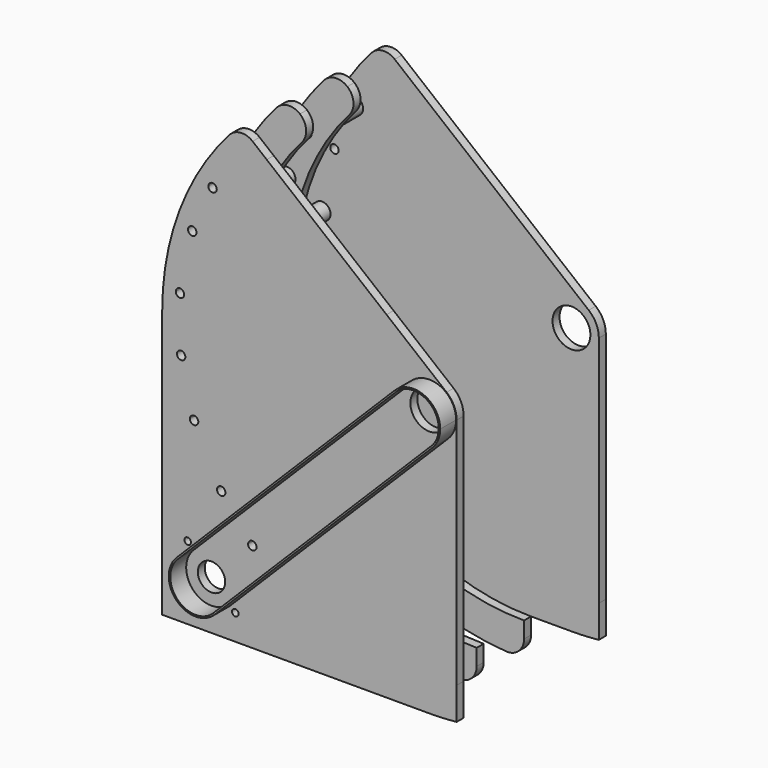
from build123d import *
from build123d import SkipClean  # not in build123d's __all__

# Parameters (mm, degrees)
F0_R      = 3.175
F0_R_2    = 2.4892
F0_R_3    = 19.1008
F0_R_4    = 10.31875
F1_DEPTH  = 6.604
F2_R      = 6.35
F3_DEPTH  = 38.1
F4_R      = 6.35
F4_R_2    = 3.175
F5_DEPTH  = 6.604
F6_R      = 6.35
F7_DEPTH  = 38.1
F8_R      = 3.175
F9_DEPTH  = 6.604
F10_R     = 6.35
F11_DEPTH = 38.1
F12_R     = 3.175
F12_R_2   = 25.4
F12_R_3   = 14.2875
F13_DEPTH = 6.604
F14_R     = 3.175
F15_DEPTH = 140.717
F16_R     = 12.69999
F18_DEPTH = 15


# Not quite as in the source:
# - a fillet or chamfer is up to 0.001 mm smaller than in the source, because OpenCascade refuses the exact size


with BuildPart() as f1:
    # F0 (on Front) → F1 (new body)
    with BuildSketch(Plane.XZ):
        with BuildLine():
            Line((20.6375, -174.9998249999), (20.6375, -58.3716647869))
            ThreePointArc((20.6375, -58.3716647869), (-52.3694193672, -33.0242573178), (-43.7787485902, 43.7787485902))
            Line((-43.7787485902, 43.7787485902), (-124.6010536798, 124.6010536798))
            ThreePointArc((-124.6010536798, 124.6010536798), (-162.7991221226, -67.4336043256), (0, -176.2125))
            ThreePointArc((0, -176.2125), (10.3365490724, -175.9090700036), (20.6375, -174.9998249999))
        make_face()
        with BuildLine():
            ThreePointArc((0, -176.2125), (-162.7991221226, -67.4336043256), (-124.6010536798, 124.6010536798))
            Line((-124.6010536798, 124.6010536798), (-142.561565922, 142.561565922))
            ThreePointArc((-142.561565922, 142.561565922), (-186.2656622484, 77.1537635077), (-201.6125, 0))
            ThreePointArc((-201.6125, 0), (-172.0465507714, -105.1074903321), (-92.0202423383, -179.3875))
            Line((-92.0202423383, -179.3875), (20.6358525902, -179.3875))
            Line((20.6358525902, -179.3875), (20.6358525902, -176.2125))
            Line((20.6358525902, -176.2125), (0, -176.2125))
        make_face()
        with Locations((-133.5813098009, -133.5813098009)):
            Circle(F0_R, mode=Mode.SUBTRACT)
        with Locations((-177.5196822242, -64.611880326)):
            Circle(F0_R, mode=Mode.SUBTRACT)
        with Locations((-188.1936309033, 16.4648092518)):
            Circle(F0_R, mode=Mode.SUBTRACT)
        with Locations((-163.6030240924, 94.45625)):
            Circle(F0_R, mode=Mode.SUBTRACT)
        with BuildLine():
            ThreePointArc((-92.0202423383, -179.3875), (-172.0465507714, -105.1074903321), (-201.6125, 0))
            Line((-201.6125, 0), (-201.6125, -201.6125))
            Line((-201.6125, -201.6125), (0, -201.6125))
            ThreePointArc((0, -201.6125), (-47.3330635629, -195.9775018975), (-92.0202423383, -179.3875))
        make_face()
        with Locations((-146.444987879, -182.3660123632)):
            Circle(F0_R_2, mode=Mode.SUBTRACT)
        with Locations((-164.4055001211, -164.4055001211)):
            Circle(F0_R_3, mode=Mode.SUBTRACT)
        with Locations((-182.3660123632, -146.444987879)):
            Circle(F0_R_2, mode=Mode.SUBTRACT)
        with BuildLine():
            ThreePointArc((-43.7787485902, 43.7787485902), (-52.3694193672, -33.0242573178), (20.6375, -58.3716647869))
            Line((20.6375, -58.3716647869), (20.6375, 0))
            ThreePointArc((20.6375, 0), (-7.8976293354, -19.0665638522), (-14.5929161967, 14.5929161967))
            Line((-14.5929161967, 14.5929161967), (-43.7787485902, 43.7787485902))
        make_face()
        with BuildLine():
            Line((20.6358525902, -179.3875), (-92.0202423383, -179.3875))
            ThreePointArc((-92.0202423383, -179.3875), (-47.3330635629, -195.9775018975), (0, -201.6125))
            ThreePointArc((0, -201.6125), (10.3315003836, -201.347610505), (20.6358525902, -200.5536380725))
            Line((20.6358525902, -200.5536380725), (20.6358525902, -179.3875))
        make_face()
        with BuildLine():
            ThreePointArc((20.6375, 0), (18.6367679163, 8.864383108), (13.0224993569, 16.0100255074))
            ThreePointArc((13.0224993569, 16.0100255074), (-1.0576398075, 20.6103809836), (-14.5929161967, 14.5929161967))
            ThreePointArc((-14.5929161967, 14.5929161967), (-7.8976293354, -19.0665638522), (20.6375, 0))
        make_face()
        with BuildLine():
            ThreePointArc((19.1008, 0), (-7.3095597049, -17.6468381746), (-13.5063052061, 13.5063052061))
            ThreePointArc((-13.5063052061, 13.5063052061), (7.3095597049, 17.6468381746), (19.1008, 0))
        make_face(mode=Mode.SUBTRACT)
        with BuildLine():
            ThreePointArc((19.1008, 0), (7.3095597049, 17.6468381746), (-13.5063052061, 13.5063052061))
            ThreePointArc((-13.5063052061, 13.5063052061), (-7.3095597049, -17.6468381746), (19.1008, 0))
        make_face()
        with BuildLine():
            ThreePointArc((14.2875, 0), (-5.4675895399, -13.1999288208), (-10.1027881362, 10.1027881362))
            ThreePointArc((-10.1027881362, 10.1027881362), (5.4675895399, 13.1999288208), (14.2875, 0))
        make_face(mode=Mode.SUBTRACT)
        with Locations((-164.4055001211, -164.4055001211)):
            Circle(F0_R_3)
        with Locations((-164.4055001211, -164.4055001211)):
            Circle(F0_R_4, mode=Mode.SUBTRACT)
        with BuildLine():
            ThreePointArc((-43.7787485902, 43.7787485902), (-38.2889048868, 48.6530309315), (-32.2606910562, 52.8432159206))
            Line((-32.2606910562, 52.8432159206), (-122.7377265448, 126.4369235582))
            ThreePointArc((-122.7377265448, 126.4369235582), (-123.6727967473, 125.5224462037), (-124.6010536798, 124.6010536798))
            Line((-124.6010536798, 124.6010536798), (-43.7787485902, 43.7787485902))
        make_face()
        with BuildLine():
            Line((13.0224993569, 16.0100255074), (-32.2606910562, 52.8432159206))
            ThreePointArc((-32.2606910562, 52.8432159206), (-38.2889048868, 48.6530309315), (-43.7787485902, 43.7787485902))
            Line((-43.7787485902, 43.7787485902), (-14.5929161967, 14.5929161967))
            ThreePointArc((-14.5929161967, 14.5929161967), (-1.0576398075, 20.6103809836), (13.0224993569, 16.0100255074))
        make_face()
        with BuildLine():
            ThreePointArc((-124.6010536798, 124.6010536798), (-123.6727967473, 125.5224462037), (-122.7377265448, 126.4369235582))
            Line((-122.7377265448, 126.4369235582), (-142.561565922, 142.561565922))
            Line((-142.561565922, 142.561565922), (-124.6010536798, 124.6010536798))
        make_face()
        with BuildLine():
            Line((20.6375, -176.2125), (20.6375, -174.9998249999))
            ThreePointArc((20.6375, -174.9998249999), (10.3365490724, -175.9090700036), (0, -176.2125))
            Line((0, -176.2125), (20.6358525902, -176.2125))
            Line((20.6358525902, -176.2125), (20.6375, -176.2125))
        make_face()
    extrude(amount=F1_DEPTH)

    # F2 (on face) → F3 (join)
    with BuildSketch(Plane(origin=(0, 0, 0), x_dir=(-1, 0, 0), z_dir=(0, 1, 0))):
        with Locations((163.6030240924, 94.45625)):
            Circle(F2_R)
        with Locations((188.1936309033, 16.4648092518)):
            Circle(F2_R)
        with Locations((177.5196822242, -64.611880326)):
            Circle(F2_R)
        with Locations((133.5813098009, -133.5813098009)):
            Circle(F2_R)
    extrude(amount=F3_DEPTH)

    # F4 (on face) → F5 (join)
    with BuildSketch(Plane(origin=(0, 38.1, 0), x_dir=(-1, 0, 0), z_dir=(0, 1, 0))):
        with BuildLine():
            ThreePointArc((0, -201.6125), (142.561565922, -142.561565922), (201.6125, 0))
            ThreePointArc((201.6125, 0), (186.2656622484, 77.1537635077), (142.561565922, 142.561565922))
            Line((142.561565922, 142.561565922), (137.5828187691, 138.5118702131))
            ThreePointArc((137.5828187691, 138.5118702131), (139.3142009541, 136.3119615594), (139.9313098009, 133.5813098009))
            ThreePointArc((139.9313098009, 133.5813098009), (135.0804626561, 127.410812194), (127.9391709925, 130.6677604763))
            Line((127.9391709925, 130.6677604763), (122.7377265448, 126.4369235582))
            ThreePointArc((122.7377265448, 126.4369235582), (162.2941261953, 68.6400885689), (176.2125, 0))
            ThreePointArc((176.2125, 0), (124.6010536798, -124.6010536798), (0, -176.2125))
            Line((0, -176.2125), (0, -201.6125))
        make_face()
        with Locations((94.45625, -163.6030240924)):
            Circle(F4_R, mode=Mode.SUBTRACT)
        with Locations((133.5813098009, -133.5813098009)):
            Circle(F4_R_2, mode=Mode.SUBTRACT)
        with Locations((157.0750031341, -104.9541616453)):
            Circle(F4_R, mode=Mode.SUBTRACT)
        with Locations((177.5196822242, -64.611880326)):
            Circle(F4_R_2, mode=Mode.SUBTRACT)
        with Locations((187.2963273743, -24.6580292878)):
            Circle(F4_R, mode=Mode.SUBTRACT)
        with Locations((188.1936309033, 16.4648092518)):
            Circle(F4_R_2, mode=Mode.SUBTRACT)
        with Locations((178.8869380882, 60.7239329891)):
            Circle(F4_R, mode=Mode.SUBTRACT)
        with Locations((163.6030240924, 94.45625)):
            Circle(F4_R, mode=Mode.SUBTRACT)
        with BuildLine():
            ThreePointArc((139.9313098009, 133.5813098009), (139.3142009541, 136.3119615594), (137.5828187691, 138.5118702131))
            Line((137.5828187691, 138.5118702131), (127.9391709925, 130.6677604763))
            ThreePointArc((127.9391709925, 130.6677604763), (135.0804626561, 127.410812194), (139.9313098009, 133.5813098009))
        make_face()
        with Locations((178.8869380882, 60.7239329891)):
            Circle(F4_R)
        with Locations((178.8869380882, 60.7239329891)):
            Circle(F4_R_2, mode=Mode.SUBTRACT)
        with Locations((187.2963273743, -24.6580292878)):
            Circle(F4_R)
        with Locations((187.2963273743, -24.6580292878)):
            Circle(F4_R_2, mode=Mode.SUBTRACT)
        with Locations((157.0750031341, -104.9541616453)):
            Circle(F4_R)
        with Locations((157.0750031341, -104.9541616453)):
            Circle(F4_R_2, mode=Mode.SUBTRACT)
        with Locations((94.45625, -163.6030240924)):
            Circle(F4_R)
        with Locations((163.6030240924, 94.45625)):
            Circle(F4_R)
        with Locations((163.6030240924, 94.45625)):
            Circle(F4_R_2, mode=Mode.SUBTRACT)
    extrude(amount=F5_DEPTH)

    # F6 (on face) → F7 (join)
    with BuildSketch(Plane(origin=(0, 44.704, 0), x_dir=(-1, 0, 0), z_dir=(0, 1, 0))):
        with Locations((178.8869380882, 60.7239329891)):
            Circle(F6_R)
        with Locations((187.2963273743, -24.6580292878)):
            Circle(F6_R)
        with Locations((157.0750031341, -104.9541616453)):
            Circle(F6_R)
    extrude(amount=F7_DEPTH)

    # F8 (on face) → F9 (join)
    with BuildSketch(Plane(origin=(0, 82.804, 0), x_dir=(-1, 0, 0), z_dir=(0, 1, 0))):
        with BuildLine():
            ThreePointArc((122.7377265448, 126.4369235582), (163.2951492678, -66.2234050912), (0, -176.2125))
            Line((0, -176.2125), (0, -201.6125))
            ThreePointArc((0, -201.6125), (186.2656622484, -77.1537635077), (142.561565922, 142.561565922))
            Line((142.561565922, 142.561565922), (122.7377265448, 126.4369235582))
        make_face()
        with Locations((133.5813098009, -133.5813098009)):
            Circle(F8_R, mode=Mode.SUBTRACT)
        with Locations((157.0750031341, -104.9541616453)):
            Circle(F8_R, mode=Mode.SUBTRACT)
        with Locations((177.5196822242, -64.611880326)):
            Circle(F8_R, mode=Mode.SUBTRACT)
        with Locations((187.2963273743, -24.6580292878)):
            Circle(F8_R, mode=Mode.SUBTRACT)
        with Locations((188.1936309033, 16.4648092518)):
            Circle(F8_R, mode=Mode.SUBTRACT)
        with Locations((163.6030240924, 94.45625)):
            Circle(F8_R, mode=Mode.SUBTRACT)
        with Locations((178.8869380882, 60.7239329891)):
            Circle(F8_R, mode=Mode.SUBTRACT)
    extrude(amount=F9_DEPTH)

    # F10 (on face) → F11 (join)
    with BuildSketch(Plane(origin=(0, 89.408, 0), x_dir=(-1, 0, 0), z_dir=(0, 1, 0))):
        with Locations((163.6030240924, 94.45625)):
            Circle(F10_R)
        with Locations((188.1936309033, 16.4648092518)):
            Circle(F10_R)
        with Locations((177.5196822242, -64.611880326)):
            Circle(F10_R)
        with Locations((133.5813098009, -133.5813098009)):
            Circle(F10_R)
    extrude(amount=F11_DEPTH)

    # F12 (on face) → F13 (join)
    with BuildSketch(Plane(origin=(0, 127.508, 0), x_dir=(-1, 0, 0), z_dir=(0, 1, 0))):
        with BuildLine():
            Line((142.561565922, 142.561565922), (-13.0224993569, 16.0100255074))
            ThreePointArc((-13.0224993569, 16.0100255074), (-18.6367679163, 8.864383108), (-20.6375, 0))
            Line((-20.6375, 0), (-20.6375, -176.2125))
            Line((-20.6375, -176.2125), (-20.6358525902, -200.5536380725))
            ThreePointArc((-20.6358525902, -200.5536380725), (-10.3315003836, -201.347610505), (0, -201.6125))
            Line((0, -201.6125), (201.6125, -201.6125))
            Line((201.6125, -201.6125), (201.6125, 0))
            ThreePointArc((201.6125, 0), (186.2656622484, 77.1537635077), (142.561565922, 142.561565922))
        make_face()
        with Locations((133.5813098009, -133.5813098009)):
            Circle(F12_R, mode=Mode.SUBTRACT)
        with Locations((164.4055001211, -164.4055001211)):
            Circle(F12_R_2, mode=Mode.SUBTRACT)
        with Locations((177.5196822242, -64.611880326)):
            Circle(F12_R, mode=Mode.SUBTRACT)
        Circle(F12_R_3, mode=Mode.SUBTRACT)
        with Locations((188.1936309033, 16.4648092518)):
            Circle(F12_R, mode=Mode.SUBTRACT)
        with Locations((163.6030240924, 94.45625)):
            Circle(F12_R, mode=Mode.SUBTRACT)
    extrude(amount=F13_DEPTH)

    # F14 (on face) → F15 (cut, through all)
    with BuildSketch(Plane(origin=(0, 134.112, 0), x_dir=(-1, 0, 0), z_dir=(0, 1, 0))):
        with Locations((163.6030240924, 94.45625)):
            Circle(F14_R)
        with Locations((188.1936309033, 16.4648092518)):
            Circle(F14_R)
        with Locations((177.5196822242, -64.611880326)):
            Circle(F14_R)
        with Locations((133.5813098009, -133.5813098009)):
            Circle(F14_R)
        with Locations((157.0750031341, -104.9541616453)):
            Circle(F14_R)
        with Locations((187.2963273743, -24.6580292878)):
            Circle(F14_R)
        with Locations((178.8869380882, 60.7239329891)):
            Circle(F14_R)
    with SkipClean():  # cleaning this boolean's faces spoils the solid; the shape is the same uncleaned
        extrude(amount=-F15_DEPTH, mode=Mode.SUBTRACT)

    # F16 (radius 12.7 in the source; OpenCascade refuses exactly that, so slightly less here)
    f16_edges = [f1.edges().sort_by_distance(p)[0] for p in [
        (-142.561566, -3.302, 142.561566),
        (-142.561566, 41.402, 142.561566),
        (-122.737727, 86.106, 126.436924),
        (-142.561566, 86.106, 142.561566),
        (-122.737727, 41.402, 126.436924),
        (-142.561566, 130.81, 142.561566),
        (0, 41.402, -201.6125),
        (0, 86.106, -201.6125),
    ]]
    fillet(f16_edges, radius=F16_R)


with BuildPart() as f18:
    # F17 (on face) → F18 (new body)
    with BuildSketch(Plane.XZ.offset(6.604)):
        with BuildLine():
            ThreePointArc((-14.314528257, 12.6465347594), (6.7609769749, 17.8642030605), (19.1008, 0))
            ThreePointArc((19.1008, 0), (17.4126317909, -7.8511664582), (12.6465347594, -14.314528257))
            Line((12.6465347594, -14.314528257), (8.6658675036, -18.2951955128))
            ThreePointArc((8.6658675036, -18.2951955128), (11.6613067569, -16.5476694178), (14.314528257, -14.314528257))
            ThreePointArc((14.314528257, -14.314528257), (18.7028324803, -7.7469668681), (20.2438, 0))
            ThreePointArc((20.2438, 0), (7.7469668681, 18.7028324803), (-14.314528257, 14.314528257))
            ThreePointArc((-14.314528257, 14.314528257), (-16.5476694178, 11.6613067569), (-18.2951955128, 8.6658675036))
            Line((-18.2951955128, 8.6658675036), (-14.314528257, 12.6465347594))
        make_face()
        with BuildLine():
            Line((-173.0713676247, -146.1103046083), (-18.2951955128, 8.6658675036))
            ThreePointArc((-18.2951955128, 8.6658675036), (-16.5476694178, 11.6613067569), (-14.314528257, 14.314528257))
            Line((-14.314528257, 14.314528257), (-178.7200283781, -150.0909718641))
            ThreePointArc((-178.7200283781, -150.0909718641), (-176.066806878, -147.8578307033), (-173.0713676247, -146.1103046083))
        make_face()
        with BuildLine():
            ThreePointArc((14.314528257, -14.314528257), (11.6613067569, -16.5476694178), (8.6658675036, -18.2951955128))
            Line((8.6658675036, -18.2951955128), (-146.1103046083, -173.0713676247))
            ThreePointArc((-146.1103046083, -173.0713676247), (-147.8578307033, -176.066806878), (-150.0909718641, -178.7200283781))
            Line((-150.0909718641, -178.7200283781), (14.314528257, -14.314528257))
        make_face()
        with BuildLine():
            Line((-177.0520348805, -150.0909718641), (-173.0713676247, -146.1103046083))
            ThreePointArc((-173.0713676247, -146.1103046083), (-176.066806878, -147.8578307033), (-178.7200283781, -150.0909718641))
            ThreePointArc((-178.7200283781, -150.0909718641), (-178.7200283781, -178.7200283781), (-150.0909718641, -178.7200283781))
            ThreePointArc((-150.0909718641, -178.7200283781), (-147.8578307033, -176.066806878), (-146.1103046083, -173.0713676247))
            Line((-146.1103046083, -173.0713676247), (-150.0909718641, -177.0520348805))
            ThreePointArc((-150.0909718641, -177.0520348805), (-177.9118053272, -177.9118053272), (-177.0520348805, -150.0909718641))
        make_face()
    extrude(amount=F18_DEPTH)


solid = Compound([f1.part, f18.part])
